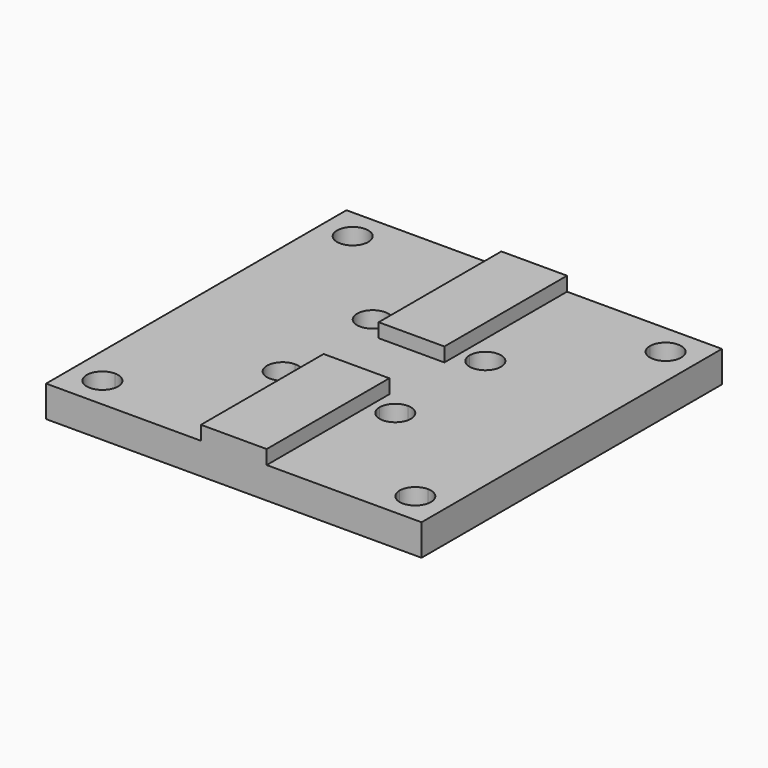
from build123d import *

# Parameters (mm, degrees)
F1_DEPTH = 5
F2_W     = 10.5
F2_H     = 24.5
F3_DEPTH = 2.25


# Not quite as in the source:
# - a feature names something its author has since deleted; it is built from what else it names


with BuildPart() as f1:
    # F0 (on Top) → F1 (new body)
    with BuildSketch(Plane.XY):
        Polygon((5.25, -30), (30, -30), (30, 30), (-30, 30), (-30, -30), (0, -30), align=None)
        with BuildLine():
            Line((22.5, -25), (-22.5, -25))
            ThreePointArc((-22.5, -25), (-26.767766953, -26.767766953), (-25, -22.5))
            Line((-25, -22.5), (-25, 22.5))
            ThreePointArc((-25, 22.5), (-26.767766953, 26.767766953), (-22.5, 25))
            Line((-22.5, 25), (22.5, 25))
            ThreePointArc((22.5, 25), (25, 27.5), (27.5, 25))
            ThreePointArc((27.5, 25), (26.767766953, 23.232233047), (25, 22.5))
            Line((25, 22.5), (25, -22.5))
            ThreePointArc((25, -22.5), (26.767766953, -23.232233047), (27.5, -25))
            ThreePointArc((27.5, -25), (25, -27.5), (22.5, -25))
        make_face(mode=Mode.SUBTRACT)
        with BuildLine():
            ThreePointArc((-25, -22.5), (-23.232233047, -23.232233047), (-22.5, -25))
            Line((-22.5, -25), (22.5, -25))
            ThreePointArc((22.5, -25), (23.232233047, -23.232233047), (25, -22.5))
            Line((25, -22.5), (25, 22.5))
            ThreePointArc((25, 22.5), (23.232233047, 23.232233047), (22.5, 25))
            Line((22.5, 25), (-22.5, 25))
            ThreePointArc((-22.5, 25), (-23.232233047, 23.232233047), (-25, 22.5))
            Line((-25, 22.5), (-25, -22.5))
        make_face()
        with BuildLine():
            Line((6.5, -9), (-6.5, -9))
            ThreePointArc((-6.5, -9), (-10.767766953, -10.767766953), (-9, -6.5))
            Line((-9, -6.5), (-9, 6.5))
            ThreePointArc((-9, 6.5), (-10.767766953, 10.767766953), (-6.5, 9))
            Line((-6.5, 9), (6.5, 9))
            ThreePointArc((6.5, 9), (9, 11.5), (11.5, 9))
            ThreePointArc((11.5, 9), (10.767766953, 7.232233047), (9, 6.5))
            Line((9, 6.5), (9, -6.5))
            ThreePointArc((9, -6.5), (10.767766953, -7.232233047), (11.5, -9))
            ThreePointArc((11.5, -9), (9, -11.5), (6.5, -9))
        make_face(mode=Mode.SUBTRACT)
        with BuildLine():
            ThreePointArc((-9, -6.5), (-7.232233047, -7.232233047), (-6.5, -9))
            Line((-6.5, -9), (6.5, -9))
            ThreePointArc((6.5, -9), (7.232233047, -7.232233047), (9, -6.5))
            Line((9, -6.5), (9, 6.5))
            ThreePointArc((9, 6.5), (7.232233047, 7.232233047), (6.5, 9))
            Line((6.5, 9), (-6.5, 9))
            ThreePointArc((-6.5, 9), (-7.232233047, 7.232233047), (-9, 6.5))
            Line((-9, 6.5), (-9, -6.5))
        make_face()
    extrude(amount=-F1_DEPTH)

    # F2 (on face) → F3 (join)
    with BuildSketch(Plane.XY):
        with Locations((0, 17.75)):
            Rectangle(F2_W, F2_H)
        with Locations((0, -17.75)):
            Rectangle(F2_W, F2_H)
    extrude(amount=F3_DEPTH)


solid = f1.part
